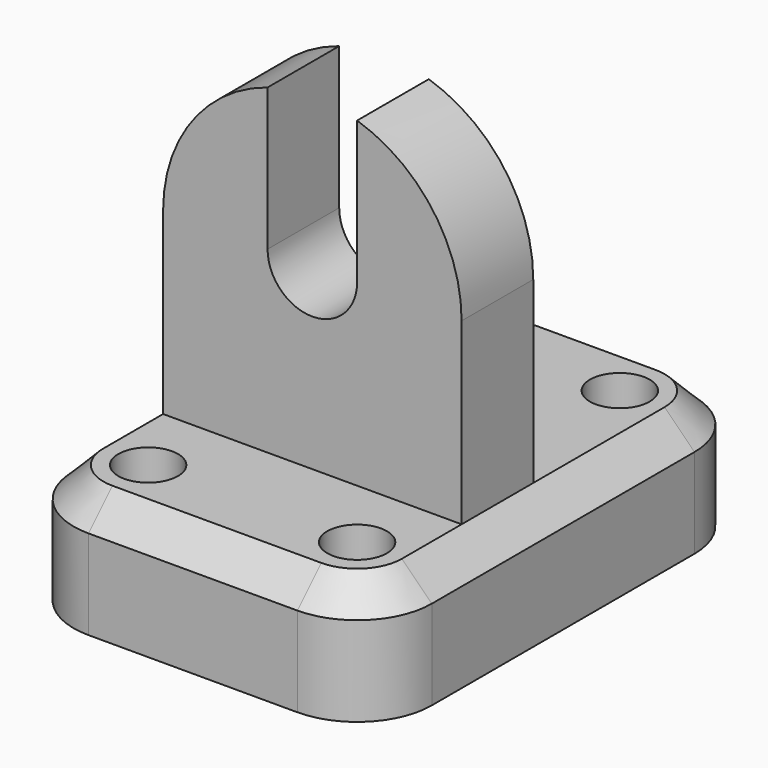
from build123d import *

# Parameters (mm, degrees)
F0_W     = 76.2
F0_H     = 101.6
F1_DEPTH = 25.4
F2_W     = 63.5
F2_H     = 19.05
F3_DEPTH = 76.2
F5_DEPTH = 54.60239
F6_DEPTH = 25.4
F8_D     = 12.7
F8_DEPTH = 215.9
F8_TIP   = 3.8154649308
F9_DEPTH = 25.4
F10_SIZE = 6.34999


# Not quite as in the source:
# - a fillet or chamfer is up to 0.001 mm smaller than in the source, because OpenCascade refuses the exact size


with BuildPart() as f1:
    # F0 (on Top) → F1 (new body)
    with BuildSketch(Plane.XY):
        with Locations((-6.5660695493, 0.5611634433)):
            Rectangle(F0_W, F0_H)
    extrude(amount=F1_DEPTH)

    # F2 (on face) → F3 (join)
    with BuildSketch(Plane.XY.offset(25.4)):
        with Locations((-6.5660695493, -8.9638365567)):
            Rectangle(F2_W, F2_H)
    extrude(amount=F3_DEPTH)

    # F4 (on face) → F5 (cut)
    with BuildSketch(Plane.XZ.offset(18.4888365567)):
        with BuildLine():
            Line((-38.3160695493, 101.6), (-38.3160695493, 63.5))
            ThreePointArc((-38.3160695493, 63.5), (-32.1637379002, 82.2835533113), (-16.0910695493, 93.787569645))
            Line((-16.0910695493, 93.787569645), (-16.0910695493, 101.6))
            Line((-16.0910695493, 101.6), (-38.3160695493, 101.6))
        make_face()
        with BuildLine():
            ThreePointArc((-16.0910695493, 93.787569645), (-6.5660695493, 95.25), (2.9589304507, 93.787569645))
            Line((2.9589304507, 93.787569645), (2.9589304507, 101.6))
            Line((2.9589304507, 101.6), (-16.0910695493, 101.6))
            Line((-16.0910695493, 101.6), (-16.0910695493, 93.787569645))
        make_face()
        with BuildLine():
            ThreePointArc((2.9589304507, 93.787569645), (19.0315988015, 82.2835533113), (25.1839304507, 63.5))
            Line((25.1839304507, 63.5), (25.1839304507, 101.6))
            Line((25.1839304507, 101.6), (2.9589304507, 101.6))
            Line((2.9589304507, 101.6), (2.9589304507, 93.787569645))
        make_face()
    extrude(amount=-F5_DEPTH, mode=Mode.SUBTRACT)

    # F4 (on face) → F6 (cut)
    with BuildSketch(Plane.XZ.offset(18.4888365567)):
        with BuildLine():
            Line((2.9589304507, 63.5), (2.9589304507, 93.787569645))
            ThreePointArc((2.9589304507, 93.787569645), (-6.5660695493, 95.25), (-16.0910695493, 93.787569645))
            Line((-16.0910695493, 93.787569645), (-16.0910695493, 63.5))
            ThreePointArc((-16.0910695493, 63.5), (-6.5660695493, 73.025), (2.9589304507, 63.5))
        make_face()
        with BuildLine():
            ThreePointArc((-16.0910695493, 63.5), (-13.3012616401, 56.7648079092), (-6.5660695493, 53.975))
            ThreePointArc((-6.5660695493, 53.975), (0.1691225415, 56.7648079092), (2.9589304507, 63.5))
            ThreePointArc((2.9589304507, 63.5), (-6.5660695493, 73.025), (-16.0910695493, 63.5))
        make_face()
    extrude(amount=-F6_DEPTH, mode=Mode.SUBTRACT)

    # F8
    with Locations(Plane.XY.offset(25.4)):
        with Locations((-28.7910695493, 35.4861634433), (15.6589304507, 35.4861634433), (15.6589304507, -34.3638365567), (-28.7910695493, -34.3638365567)):
            Hole(F8_D / 2, depth=F8_DEPTH)
            with Locations((0, 0, -(F8_DEPTH + F8_TIP / 2))):  # 118° drill point
                Cone(0, F8_D / 2, F8_TIP, mode=Mode.SUBTRACT)

    # F7 (on face) → F9 (cut)
    with BuildSketch(Plane.XY.offset(25.4)):
        with BuildLine():
            ThreePointArc((-44.6660695493, 35.4861634433), (-40.0163896548, 46.7114836405), (-28.7910694197, 51.3611634433))
            Line((-28.7910694197, 51.3611634433), (-44.6660695493, 51.3611634433))
            Line((-44.6660695493, 51.3611634433), (-44.6660695493, 35.4861634433))
        make_face()
        with BuildLine():
            Line((31.5339304507, 51.3611634433), (15.6589304507, 51.3611634433))
            ThreePointArc((15.6589304507, 51.3611634433), (26.884250602, 46.7114835947), (31.5339304507, 35.4861634433))
            Line((31.5339304507, 35.4861634433), (31.5339304507, 51.3611634433))
        make_face()
        with BuildLine():
            Line((31.5339304507, -50.2388365567), (31.5339304507, -34.3638365567))
            ThreePointArc((31.5339304507, -34.3638365567), (26.8842505737, -45.5891567363), (15.6589303706, -50.2388365567))
            Line((15.6589303706, -50.2388365567), (31.5339304507, -50.2388365567))
        make_face()
        with BuildLine():
            ThreePointArc((-28.7910695493, -50.2388365567), (-40.0163897007, -45.589156708), (-44.6660695493, -34.3638365567))
            Line((-44.6660695493, -34.3638365567), (-44.6660695493, -50.2388365567))
            Line((-44.6660695493, -50.2388365567), (-28.7910695493, -50.2388365567))
        make_face()
    extrude(amount=-F9_DEPTH, mode=Mode.SUBTRACT)

    # F10 (size 6.35 in the source; OpenCascade refuses exactly that, so slightly less here)
    f10_edges = [f1.edges().sort_by_distance(p)[0] for p in [
        (26.884251, -45.589157, 25.4),
        (31.53393, 0.561163, 25.4),
        (26.884251, 46.711484, 25.4),
        (-6.566069, 51.361163, 25.4),
        (-40.01639, 46.711484, 25.4),
        (-44.66607, 0.561163, 25.4),
        (-40.01639, -45.589157, 25.4),
        (-6.56607, -50.238837, 25.4),
    ]]
    chamfer(f10_edges, length=F10_SIZE)


solid = f1.part
